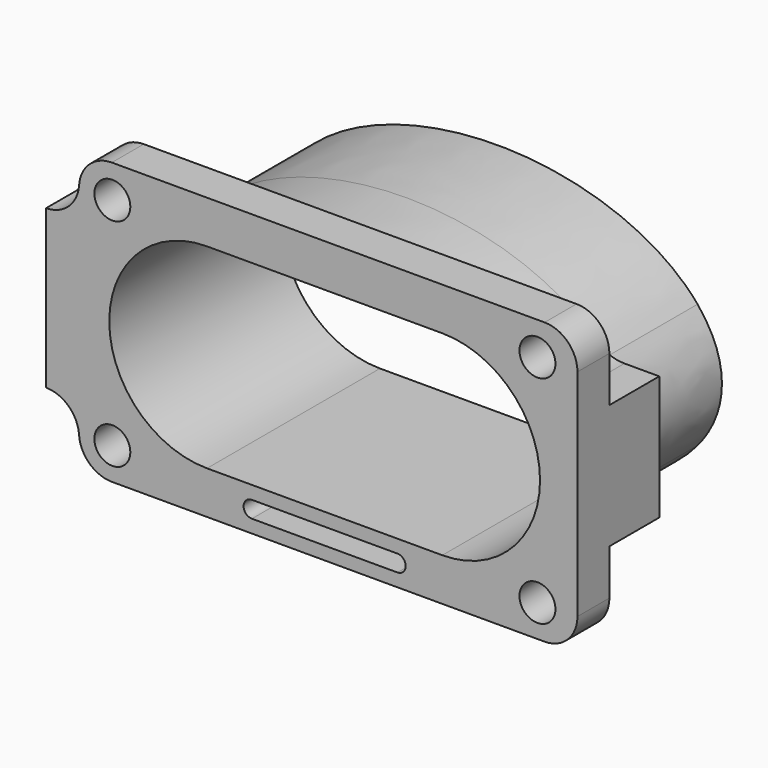
from build123d import *

# Parameters (mm, degrees)
F0_R        = 5.4864
F1_DEPTH    = 12.192
F3_DEPTH    = 19.05
F5_DEPTH    = 34.798
F6_R        = 10.033
F7_T4_DEPTH = 12.192
F7_T9_DEPTH = 12.192
F8_R        = 12.7
F10_DEPTH   = 25.4


# Not quite as in the source:
# - a fillet or chamfer that OpenCascade refuses, or shapes differently, is made with other operations: its cross-section is extruded or revolved along the edge and cut away or added


with BuildPart() as f1:
    # F0 (on Front) → F1 (new body)
    with BuildSketch(Plane.XZ):
        Polygon((-75.0316, 24.13), (-85.09, 24.13), (-85.09, -24.13), (-75.0316, -24.13), (-75.0316, -42.926), (77.216, -42.926), (77.216, 42.926), (-75.0316, 42.926), align=None)
        with Locations((-64.8462, -33.1216)):
            Circle(F0_R, mode=Mode.SUBTRACT)
        with Locations((64.9986, -33.1216)):
            Circle(F0_R, mode=Mode.SUBTRACT)
        with Locations((-64.8462, 32.8676)):
            Circle(F0_R, mode=Mode.SUBTRACT)
        with BuildLine():
            Line((35.941, -29.845), (-35.941, -29.845))
            ThreePointArc((-35.941, -29.845), (-65.786, 0), (-35.941, 29.845))
            Line((-35.941, 29.845), (35.941, 29.845))
            ThreePointArc((35.941, 29.845), (65.786, 0), (35.941, -29.845))
        make_face(mode=Mode.SUBTRACT)
        with Locations((64.9986, 32.8676)):
            Circle(F0_R, mode=Mode.SUBTRACT)
    extrude(amount=-F1_DEPTH)

    # F2 (on face) → F3 (join)
    with BuildSketch(Plane(origin=(0, 12.192, 0), x_dir=(-1, 0, 0), z_dir=(0, 1, 0))):
        with BuildLine():
            add(Edge.make_bspline(
                [(-61.0821252186, 18.9865), (-68.5165, 10.0378265977), (-68.5165, 0)],
                knots=[5.8130237676, 5.8130237676, 5.8130237676, 6.2831853072, 6.2831853072, 6.2831853072], degree=2, weights=[1, 0.9724955315, 1]))
            add(Edge.make_bspline(
                [(-68.5165, 0), (-68.5165, -10.0378265977), (-61.0821252186, -18.9865)],
                knots=[0, 0, 0, 0.4701615396, 0.4701615396, 0.4701615396], degree=2, weights=[1, 0.9724955315, 1]))
            add(Edge.make_bspline(
                [(-61.0821252186, -18.9865), (-9.5155823774, -81.056568289), (56.0204921364, -24.13)],
                knots=[0.4701615396, 0.4701615396, 0.4701615396, 2.5280622458, 2.5280622458, 2.5280622458], degree=2, weights=[1, 0.5157184224, 1]))
            add(Edge.make_bspline(
                [(56.0204921364, -24.13), (83.7998845283, 0), (56.0204921364, 24.13)],
                knots=[2.5280622458, 2.5280622458, 2.5280622458, 3.7551230613, 3.7551230613, 3.7551230613], degree=2, weights=[1, 0.8176204584, 1]))
            add(Edge.make_bspline(
                [(56.0204921364, 24.13), (-9.5155823774, 81.056568289), (-61.0821252186, 18.9865)],
                knots=[3.7551230613, 3.7551230613, 3.7551230613, 5.8130237676, 5.8130237676, 5.8130237676], degree=2, weights=[1, 0.5157184224, 1]))
        make_face()
        with BuildLine():
            ThreePointArc((35.941, 29.845), (65.786, 0), (35.941, -29.845))
            Line((35.941, -29.845), (-35.941, -29.845))
            ThreePointArc((-35.941, -29.845), (-65.786, 0), (-35.941, 29.845))
            Line((-35.941, 29.845), (35.941, 29.845))
        make_face(mode=Mode.SUBTRACT)
        with BuildLine():
            add(Edge.make_bspline(
                [(-68.5165, 0), (-68.5165, -10.0378265977), (-61.0821252186, -18.9865)],
                knots=[0, 0, 0, 0.4701615396, 0.4701615396, 0.4701615396], degree=2, weights=[1, 0.9724955315, 1]))
            add(Edge.make_bspline(
                [(-61.0821252186, 18.9865), (-68.5165, 10.0378265977), (-68.5165, 0)],
                knots=[5.8130237676, 5.8130237676, 5.8130237676, 6.2831853072, 6.2831853072, 6.2831853072], degree=2, weights=[1, 0.9724955315, 1]))
            Line((-61.0821252186, 18.9865), (-77.216, 18.9865))
            Line((-77.216, 18.9865), (-77.216, -18.9865))
            Line((-77.216, -18.9865), (-61.0821252186, -18.9865))
        make_face()
        with BuildLine():
            add(Edge.make_bspline(
                [(56.0204921364, -24.13), (83.7998845283, 0), (56.0204921364, 24.13)],
                knots=[2.5280622458, 2.5280622458, 2.5280622458, 3.7551230613, 3.7551230613, 3.7551230613], degree=2, weights=[1, 0.8176204584, 1]))
            Line((56.0204921364, -24.13), (85.09, -24.13))
            Line((85.09, -24.13), (85.09, 24.13))
            Line((85.09, 24.13), (56.0204921364, 24.13))
        make_face()
    extrude(amount=F3_DEPTH)

    # F4 (on face) → F5 (join)
    with BuildSketch(Plane(origin=(0, 31.242, 0), x_dir=(-1, 0, 0), z_dir=(0, 1, 0))):
        with BuildLine():
            add(Edge.make_bspline(
                [(-61.0821252186, 18.9865), (-68.5165, 10.0378265977), (-68.5165, 0)],
                knots=[5.8130237676, 5.8130237676, 5.8130237676, 6.2831853072, 6.2831853072, 6.2831853072], degree=2, weights=[1, 0.9724955315, 1]))
            add(Edge.make_bspline(
                [(-68.5165, 0), (-68.5165, -10.0378265977), (-61.0821252186, -18.9865)],
                knots=[0, 0, 0, 0.4701615396, 0.4701615396, 0.4701615396], degree=2, weights=[1, 0.9724955315, 1]))
            add(Edge.make_bspline(
                [(-61.0821252186, -18.9865), (-9.5155823774, -81.056568289), (56.0204921364, -24.13)],
                knots=[0.4701615396, 0.4701615396, 0.4701615396, 2.5280622458, 2.5280622458, 2.5280622458], degree=2, weights=[1, 0.5157184224, 1]))
            add(Edge.make_bspline(
                [(56.0204921364, -24.13), (83.7998845283, 0), (56.0204921364, 24.13)],
                knots=[2.5280622458, 2.5280622458, 2.5280622458, 3.7551230613, 3.7551230613, 3.7551230613], degree=2, weights=[1, 0.8176204584, 1]))
            add(Edge.make_bspline(
                [(56.0204921364, 24.13), (-9.5155823774, 81.056568289), (-61.0821252186, 18.9865)],
                knots=[3.7551230613, 3.7551230613, 3.7551230613, 5.8130237676, 5.8130237676, 5.8130237676], degree=2, weights=[1, 0.5157184224, 1]))
        make_face()
        with BuildLine():
            Line((-35.941, 29.845), (35.941, 29.845))
            ThreePointArc((35.941, 29.845), (65.786, 0), (35.941, -29.845))
            Line((35.941, -29.845), (-35.941, -29.845))
            ThreePointArc((-35.941, -29.845), (-65.786, 0), (-35.941, 29.845))
        make_face(mode=Mode.SUBTRACT)
    extrude(amount=F5_DEPTH)

    # F6
    f6_edges = [f1.edges().sort_by_distance(p)[0] for p in [
        (-75.0316, 6.096, 42.926),
        (77.216, 6.096, 42.926),
        (77.216, 6.096, -42.926),
        (-75.0316, 6.096, -42.926),
    ]]
    fillet(f6_edges, radius=F6_R)

    # F7: fillet of radius 10.16 on 2 edges, made by hand


with BuildPart() as f7_tool2:
    # F7_s3 → F7_t4 (new body)
    with BuildSketch(Plane.XZ):
        with BuildLine():
            ThreePointArc((-85.1432181398, -24.13), (-78.2119770428, -26.8614404589), (-75.0075612141, -33.5871069182))
            Line((-75.0075612141, -33.5871069182), (-73.9939955216, -33.5168176101))
            ThreePointArc((-73.9939955216, -33.5168176101), (-74.0156, -32.893), (-74.0156, -24.13))
            Line((-74.0156, -24.13), (-75.0316, -23.114))
            Line((-75.0316, -23.114), (-85.1432181398, -23.114))
            Line((-85.1432181398, -23.114), (-85.1432181398, -24.13))
        make_face()
    extrude(amount=-F7_T4_DEPTH)

    split(bisect_by=Plane.YZ.offset(-85.09), keep=Keep.TOP)


with BuildPart() as f1_1:
    add(f1.part)

    # F7_t1: union F7_tool2
    add(f7_tool2.part)


with BuildPart() as f7_tool7:
    # F7_s8 → F7_t9 (new body)
    with BuildSketch(Plane.XZ):
        with BuildLine():
            ThreePointArc((-75.0075612141, 33.5871069182), (-78.2119770428, 26.8614404589), (-85.1432181398, 24.13))
            Line((-85.1432181398, 24.13), (-85.1432181398, 23.114))
            Line((-85.1432181398, 23.114), (-75.0316, 23.114))
            Line((-75.0316, 23.114), (-74.0156, 24.13))
            ThreePointArc((-74.0156, 24.13), (-74.0156, 32.893), (-73.9939955216, 33.5168176101))
            Line((-73.9939955216, 33.5168176101), (-75.0075612141, 33.5871069182))
        make_face()
    extrude(amount=-F7_T9_DEPTH)

    split(bisect_by=Plane.YZ.offset(-85.09), keep=Keep.TOP)


with BuildPart() as f1_2:
    add(f1_1.part)

    # F7_t6: union F7_tool7
    add(f7_tool7.part)

    # F8 (call 1 of 4: OpenCascade refuses the feature's edges together)
    f8_edges = [f1_2.edges().sort_by_distance(p)[0] for p in [
        (-56.020492, 21.717, 24.13),
    ]]
    fillet(f8_edges, radius=F8_R)

    # F8#3 (call 2 of 4)
    f8_3_edges = [f1_2.edges().sort_by_distance(p)[0] for p in [
        (61.082125, 21.717, -18.9865),
    ]]
    fillet(f8_3_edges, radius=F8_R)

    # F8#4 (call 3 of 4)
    f8_4_edges = [f1_2.edges().sort_by_distance(p)[0] for p in [
        (-56.020492, 21.717, -24.13),
    ]]
    fillet(f8_4_edges, radius=F8_R)

    # F8#2 (call 4 of 4)
    f8_2_edges = [f1_2.edges().sort_by_distance(p)[0] for p in [
        (61.082125, 21.717, 18.9865),
    ]]
    fillet(f8_2_edges, radius=F8_R)

    # F9 (on face) → F10 (cut)
    with BuildSketch(Plane.XZ):
        with BuildLine():
            ThreePointArc((22.225, -38.9382), (24.765, -36.3982), (22.225, -33.8582))
            Line((22.225, -33.8582), (-22.225, -33.8582))
            ThreePointArc((-22.225, -33.8582), (-24.765, -36.3982), (-22.225, -38.9382))
            Line((-22.225, -38.9382), (22.225, -38.9382))
        make_face()
    extrude(amount=-F10_DEPTH, mode=Mode.SUBTRACT)


solid = f1_2.part
